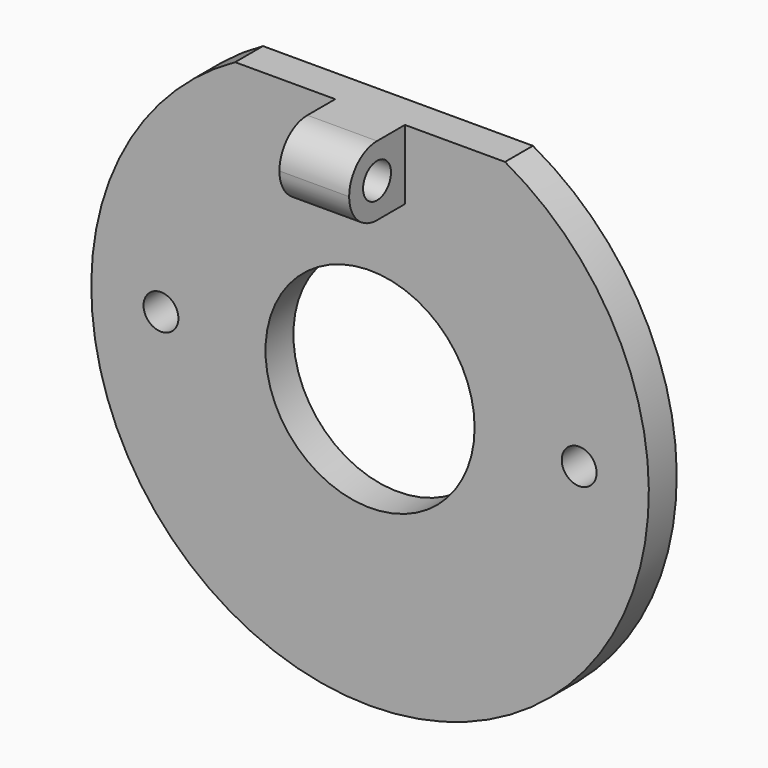
from build123d import *

# Parameters (mm, degrees)
F0_R      = 50.8
F1_DEPTH  = 6.35
F2_W      = 12.7
F2_H      = 12.7
F3_DEPTH  = 12.7
F4_R      = 6.34999
F5_R      = 3.175
F6_DEPTH  = 57.151
F7_R      = 3.175
F7_R_2    = 19.05
F8_DEPTH  = 6.351
F10_DEPTH = 6.351


# Not quite as in the source:
# - a fillet or chamfer is up to 0.001 mm smaller than in the source, because OpenCascade refuses the exact size


with BuildPart() as f1:
    # F0 (on Front) → F1 (new body)
    with BuildSketch(Plane.XZ):
        Circle(F0_R)
    extrude(amount=F1_DEPTH)

    # F2 (on face) → F3 (join)
    with BuildSketch(Plane.XZ.offset(6.35)):
        with Locations((0, 38.1)):
            Rectangle(F2_W, F2_H)
    extrude(amount=F3_DEPTH)

    # F4 (radius 6.35 in the source; OpenCascade refuses exactly that, so slightly less here)
    f4_edges = [f1.edges().sort_by_distance(p)[0] for p in [
        (0, -19.05, 31.75),
        (0, -19.05, 44.45),
    ]]
    fillet(f4_edges, radius=F4_R)

    # F5 (on face) → F6 (cut, through all)
    with BuildSketch(Plane(origin=(-6.35, 0, 0), x_dir=(0, -1, 0), z_dir=(-1, 0, 0))):
        with Locations((12.7, 38.1)):
            Circle(F5_R)
    extrude(amount=-F6_DEPTH, mode=Mode.SUBTRACT)

    # F7 (on face) → F8 (cut, through all)
    with BuildSketch(Plane.XZ.offset(6.35)):
        with Locations((-38.1, 0)):
            Circle(F7_R)
        with Locations((38.1, 0)):
            Circle(F7_R)
        Circle(F7_R_2)
    extrude(amount=-F8_DEPTH, mode=Mode.SUBTRACT)

    # F9 (on face) → F10 (cut, through all)
    with BuildSketch(Plane.XZ.offset(6.35)):
        with BuildLine():
            Line((-24.5934442484, 44.45), (6.35, 44.45))
            Line((6.35, 44.45), (24.5934442484, 44.45))
            ThreePointArc((24.5934442484, 44.45), (0, 50.8), (-24.5934442484, 44.45))
        make_face()
    extrude(amount=-F10_DEPTH, mode=Mode.SUBTRACT)


solid = f1.part
